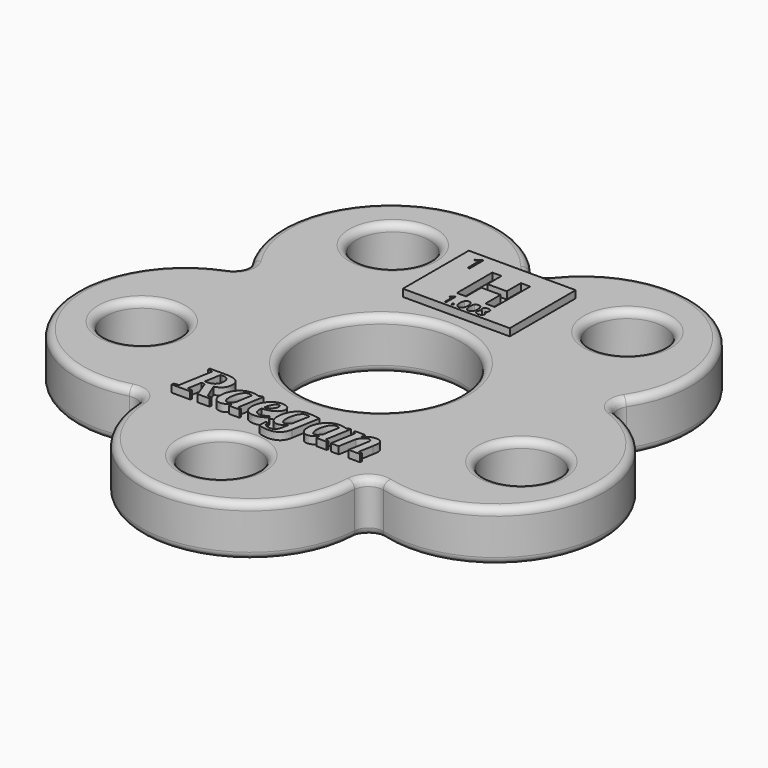
from build123d import *

# Parameters (mm, degrees)
F0_R         = 5
F0_R_2       = 11
F1_DEPTH     = 7
F2_R         = 2
F3_R         = 1
F4_W         = 14.733908698
F4_H         = 11.3537767902
F4_TEXT_SIZE = 8.3333333333
F5_DEPTH     = 1


# Not quite as in the source:
# - Text() gives the source's letters only with a copy of the font that has no kerning and outlines rounded to 1/6400 em; it was checked with that copy


with BuildPart() as f1:
    # F0 (on Top) → F1 (new body)
    with BuildSketch(Plane.XY):
        with BuildLine():
            ThreePointArc((24.0433357957, 7.8121533632), (22.041946961, 30.3381372891), (0, 25.2806593338))
            ThreePointArc((0, 25.2806593338), (-22.041946961, 30.3381372891), (-24.0433357957, 7.8121533632))
            ThreePointArc((-24.0433357957, 7.8121533632), (-35.6646193611, -11.5881372891), (-14.8595987247, -20.4524830301))
            ThreePointArc((-14.8595987247, -20.4524830301), (0, -37.5), (14.8595987247, -20.4524830301))
            ThreePointArc((14.8595987247, -20.4524830301), (35.6646193611, -11.5881372891), (24.0433357957, 7.8121533632))
        make_face()
        with Locations((-26.1540541981, -8.4979673453)):
            Circle(F0_R, mode=Mode.SUBTRACT)
        with Locations((0, -27.5)):
            Circle(F0_R, mode=Mode.SUBTRACT)
        with Locations((26.1540541981, -8.4979673453)):
            Circle(F0_R, mode=Mode.SUBTRACT)
        with Locations((-16.164094438, 22.2479673453)):
            Circle(F0_R, mode=Mode.SUBTRACT)
        Circle(F0_R_2, mode=Mode.SUBTRACT)
        with Locations((16.164094438, 22.2479673453)):
            Circle(F0_R, mode=Mode.SUBTRACT)
    extrude(amount=F1_DEPTH)

    # F2
    f2_edges = [f1.edges().sort_by_distance(p)[0] for p in [
        (14.859599, -20.452483, 3.5),
        (24.043336, 7.812153, 3.5),
        (0, 25.280659, 3.5),
        (-24.043336, 7.812153, 3.5),
        (-14.859599, -20.452483, 3.5),
    ]]
    fillet(f2_edges, radius=F2_R)

    # F3
    f3_edges = [f1.edges().sort_by_distance(p)[0] for p in [
        (35.664619, -11.588137, 7),
        (15.802257, -21.749941, 7),
        (25.568589, 8.307738, 7),
        (0, -37.5, 7),
        (22.041947, 30.338137, 7),
        (-15.802257, -21.749941, 7),
        (0, 26.884405, 7),
        (-35.664619, -11.588137, 7),
        (-22.041947, 30.338137, 7),
        (-25.568589, 8.307738, 7),
        (-31.154054, -8.497967, 7),
        (-5, -27.5, 7),
        (21.154054, -8.497967, 7),
        (-21.164094, 22.247967, 7),
        (-11, 0, 7),
        (11.164094, 22.247967, 7),
        (35.664619, -11.588137, 0),
        (15.802257, -21.749941, 0),
        (25.568589, 8.307738, 0),
        (0, -37.5, 0),
        (22.041947, 30.338137, 0),
        (-15.802257, -21.749941, 0),
        (0, 26.884405, 0),
        (-35.664619, -11.588137, 0),
        (-22.041947, 30.338137, 0),
        (-25.568589, 8.307738, 0),
        (-31.154054, -8.497967, 0),
        (-5, -27.5, 0),
        (21.154054, -8.497967, 0),
        (-21.164094, 22.247967, 0),
        (-11, 0, 0),
        (11.164094, 22.247967, 0),
    ]]
    fillet(f3_edges, radius=F3_R)

    # F4 (on face) → F5 (join)
    with BuildSketch(Plane.XY.offset(7)):
        with Locations((-0.4162131809, 19.1815658472)):
            Rectangle(F4_W, F4_H)
        with BuildLine():
            Line((-2.1715380596, 15.5983065148), (-2.1715380596, 13.9384558424))
            Line((-2.1715380596, 13.9384558424), (-2.3553604365, 13.9384558424))
            Line((-2.3553604365, 13.9384558424), (-2.3553604365, 15.1213128766))
            add(Edge.make_bspline(
                [(-2.3553604365, 15.1213128766), (-2.3553604365, 15.2691700059), (-2.3462783033, 15.4006792954)],
                knots=[0, 0, 0, 1, 1, 1], degree=2))
            add(Edge.make_bspline(
                [(-2.3462783033, 15.4006792954), (-2.3698918497, 15.3767024636), (-2.3994996041, 15.3507275625)],
                knots=[0, 0, 0, 1, 1, 1], degree=2))
            add(Edge.make_bspline(
                [(-2.3994996041, 15.3507275625), (-2.4291073585, 15.3247526614), (-2.6696022469, 15.1293051539)],
                knots=[0, 0, 0, 1, 1, 1], degree=2))
            Line((-2.6696022469, 15.1293051539), (-2.7695057126, 15.2586347314))
            Line((-2.7695057126, 15.2586347314), (-2.3302937488, 15.5983065148))
            Line((-2.3302937488, 15.5983065148), (-2.1715380596, 15.5983065148))
        make_face(mode=Mode.SUBTRACT)
        with BuildLine():
            add(Edge.make_bspline(
                [(-1.4433326158, 13.9411804824), (-1.4812959327, 13.9769640874), (-1.4812959327, 14.0587032866)],
                knots=[0, 0, 0, 1, 1, 1], degree=2))
            add(Edge.make_bspline(
                [(-1.4812959327, 14.0587032866), (-1.4812959327, 14.1349932059), (-1.4466021837, 14.1740463789)],
                knots=[0, 0, 0, 1, 1, 1], degree=2))
            add(Edge.make_bspline(
                [(-1.4466021837, 14.1740463789), (-1.4119084347, 14.2130995519), (-1.347243646, 14.2130995519)],
                knots=[0, 0, 0, 1, 1, 1], degree=2))
            add(Edge.make_bspline(
                [(-1.347243646, 14.2130995519), (-1.2814890013, 14.2130995519), (-1.2446155403, 14.1740463789)],
                knots=[0, 0, 0, 1, 1, 1], degree=2))
            add(Edge.make_bspline(
                [(-1.2446155403, 14.1740463789), (-1.2077420793, 14.1349932059), (-1.2077420793, 14.0587032866)],
                knots=[0, 0, 0, 1, 1, 1], degree=2))
            add(Edge.make_bspline(
                [(-1.2077420793, 14.0587032866), (-1.2077420793, 13.9849563647), (-1.2451604683, 13.945176621)],
                knots=[0, 0, 0, 1, 1, 1], degree=2))
            add(Edge.make_bspline(
                [(-1.2451604683, 13.945176621), (-1.2825788573, 13.9053968774), (-1.347243646, 13.9053968774)],
                knots=[0, 0, 0, 1, 1, 1], degree=2))
            add(Edge.make_bspline(
                [(-1.347243646, 13.9053968774), (-1.4053692988, 13.9053968774), (-1.4433326158, 13.9411804824)],
                knots=[0, 0, 0, 1, 1, 1], degree=2))
        make_face(mode=Mode.SUBTRACT)
        with BuildLine():
            add(Edge.make_bspline(
                [(0.0383266023, 15.405220362), (0.1785547397, 15.1859776654), (0.1785547397, 14.7707425333)],
                knots=[0, 0, 0, 1, 1, 1], degree=2))
            add(Edge.make_bspline(
                [(0.1785547397, 14.7707425333), (0.1785547397, 14.3402494173), (0.0428676689, 14.127909142)],
                knots=[0, 0, 0, 1, 1, 1], degree=2))
            add(Edge.make_bspline(
                [(0.0428676689, 14.127909142), (-0.0928194018, 13.9155688667), (-0.3721858205, 13.9155688667)],
                knots=[0, 0, 0, 1, 1, 1], degree=2))
            add(Edge.make_bspline(
                [(-0.3721858205, 13.9155688667), (-0.6399271086, 13.9155688667), (-0.779610318, 14.1329951366)],
                knots=[0, 0, 0, 1, 1, 1], degree=2))
            add(Edge.make_bspline(
                [(-0.779610318, 14.1329951366), (-0.9192935274, 14.3504214066), (-0.9192935274, 14.7707425333)],
                knots=[0, 0, 0, 1, 1, 1], degree=2))
            add(Edge.make_bspline(
                [(-0.9192935274, 14.7707425333), (-0.9192935274, 15.2041419319), (-0.7841513846, 15.4143024952)],
                knots=[0, 0, 0, 1, 1, 1], degree=2))
            add(Edge.make_bspline(
                [(-0.7841513846, 15.4143024952), (-0.6490092419, 15.6244630586), (-0.3721858205, 15.6244630586)],
                knots=[0, 0, 0, 1, 1, 1], degree=2))
            add(Edge.make_bspline(
                [(-0.3721858205, 15.6244630586), (-0.101901535, 15.6244630586), (0.0383266023, 15.405220362)],
                knots=[0, 0, 0, 1, 1, 1], degree=2))
        make_face(mode=Mode.SUBTRACT)
        with BuildLine():
            Line((-5.1220975915, 24.0717205949), (-5.1220975915, 21.6852203012))
            Line((-5.1220975915, 21.6852203012), (-5.3863937501, 21.6852203012))
            Line((-5.3863937501, 21.6852203012), (-5.3863937501, 23.385908626))
            add(Edge.make_bspline(
                [(-5.3863937501, 23.385908626), (-5.3863937501, 23.5984946667), (-5.3733356395, 23.7875761082)],
                knots=[0, 0, 0, 1, 1, 1], degree=2))
            add(Edge.make_bspline(
                [(-5.3733356395, 23.7875761082), (-5.4072867271, 23.7531026962), (-5.4498561676, 23.7157564999)],
                knots=[0, 0, 0, 1, 1, 1], degree=2))
            add(Edge.make_bspline(
                [(-5.4498561676, 23.7157564999), (-5.4924256082, 23.6784103035), (-5.8382043769, 23.3973997634)],
                knots=[0, 0, 0, 1, 1, 1], degree=2))
            Line((-5.8382043769, 23.3973997634), (-5.9818435936, 23.5833472584))
            Line((-5.9818435936, 23.5833472584), (-5.3503533648, 24.0717205949))
            Line((-5.3503533648, 24.0717205949), (-5.1220975915, 24.0717205949))
        make_face(mode=Mode.SUBTRACT)
        with BuildLine():
            add(Edge.make_bspline(
                [(1.3675876245, 15.405220362), (1.5078157618, 15.1859776654), (1.5078157618, 14.7707425333)],
                knots=[0, 0, 0, 1, 1, 1], degree=2))
            add(Edge.make_bspline(
                [(1.5078157618, 14.7707425333), (1.5078157618, 14.3402494173), (1.3721286911, 14.127909142)],
                knots=[0, 0, 0, 1, 1, 1], degree=2))
            add(Edge.make_bspline(
                [(1.3721286911, 14.127909142), (1.2364416204, 13.9155688667), (0.9570752017, 13.9155688667)],
                knots=[0, 0, 0, 1, 1, 1], degree=2))
            add(Edge.make_bspline(
                [(0.9570752017, 13.9155688667), (0.6893339135, 13.9155688667), (0.5496507042, 14.1329951366)],
                knots=[0, 0, 0, 1, 1, 1], degree=2))
            add(Edge.make_bspline(
                [(0.5496507042, 14.1329951366), (0.4099674948, 14.3504214066), (0.4099674948, 14.7707425333)],
                knots=[0, 0, 0, 1, 1, 1], degree=2))
            add(Edge.make_bspline(
                [(0.4099674948, 14.7707425333), (0.4099674948, 15.2041419319), (0.5451096375, 15.4143024952)],
                knots=[0, 0, 0, 1, 1, 1], degree=2))
            add(Edge.make_bspline(
                [(0.5451096375, 15.4143024952), (0.6802517803, 15.6244630586), (0.9570752017, 15.6244630586)],
                knots=[0, 0, 0, 1, 1, 1], degree=2))
            add(Edge.make_bspline(
                [(0.9570752017, 15.6244630586), (1.2273594871, 15.6244630586), (1.3675876245, 15.405220362)],
                knots=[0, 0, 0, 1, 1, 1], degree=2))
        make_face(mode=Mode.SUBTRACT)
        with BuildLine():
            add(Edge.make_bspline(
                [(1.9292267445, 15.5147508889), (2.0625524606, 15.6219200613), (2.2863362238, 15.6219200613)],
                knots=[0, 0, 0, 1, 1, 1], degree=2))
            add(Edge.make_bspline(
                [(2.2863362238, 15.6219200613), (2.513389555, 15.6219200613), (2.6461703431, 15.5163856729)],
                knots=[0, 0, 0, 1, 1, 1], degree=2))
            add(Edge.make_bspline(
                [(2.6461703431, 15.5163856729), (2.7789511312, 15.4108512846), (2.7789511312, 15.2248491957)],
                knots=[0, 0, 0, 1, 1, 1], degree=2))
            add(Edge.make_bspline(
                [(2.7789511312, 15.2248491957), (2.7789511312, 15.1020587542), (2.7030244972, 15.0010654324)],
                knots=[0, 0, 0, 1, 1, 1], degree=2))
            add(Edge.make_bspline(
                [(2.7030244972, 15.0010654324), (2.6270978633, 14.9000721107), (2.4599866115, 14.8172430555)],
                knots=[0, 0, 0, 1, 1, 1], degree=2))
            add(Edge.make_bspline(
                [(2.4599866115, 14.8172430555), (2.661973255, 14.7206091577), (2.7471636648, 14.6145298414)],
                knots=[0, 0, 0, 1, 1, 1], degree=2))
            add(Edge.make_bspline(
                [(2.7471636648, 14.6145298414), (2.8323540747, 14.5084505251), (2.8323540747, 14.3685856731)],
                knots=[0, 0, 0, 1, 1, 1], degree=2))
            add(Edge.make_bspline(
                [(2.8323540747, 14.3685856731), (2.8323540747, 14.1622396057), (2.6881297987, 14.0389042362)],
                knots=[0, 0, 0, 1, 1, 1], degree=2))
            add(Edge.make_bspline(
                [(2.6881297987, 14.0389042362), (2.5439055227, 13.9155688667), (2.2932386451, 13.9155688667)],
                knots=[0, 0, 0, 1, 1, 1], degree=2))
            add(Edge.make_bspline(
                [(2.2932386451, 13.9155688667), (2.0276770689, 13.9155688667), (1.8845426489, 14.0320018149)],
                knots=[0, 0, 0, 1, 1, 1], degree=2))
            add(Edge.make_bspline(
                [(1.8845426489, 14.0320018149), (1.741408229, 14.1484347631), (1.741408229, 14.3620465371)],
                knots=[0, 0, 0, 1, 1, 1], degree=2))
            add(Edge.make_bspline(
                [(1.741408229, 14.3620465371), (1.741408229, 14.6468622358), (2.0887090044, 14.8059812103)],
                knots=[0, 0, 0, 1, 1, 1], degree=2))
            add(Edge.make_bspline(
                [(2.0887090044, 14.8059812103), (1.9321330272, 14.8942595454), (1.8640170278, 14.9970692938)],
                knots=[0, 0, 0, 1, 1, 1], degree=2))
            add(Edge.make_bspline(
                [(1.8640170278, 14.9970692938), (1.7959010284, 15.0998790422), (1.7959010284, 15.2270289077)],
                knots=[0, 0, 0, 1, 1, 1], degree=2))
            add(Edge.make_bspline(
                [(1.7959010284, 15.2270289077), (1.7959010284, 15.4075817166), (1.9292267445, 15.5147508889)],
                knots=[0, 0, 0, 1, 1, 1], degree=2))
        make_face(mode=Mode.SUBTRACT)
        Polygon((2.5982840531, 16.3463894278), (1.3195982261, 16.3463894278), (1.3195982261, 18.9647829652), (-1.3417880018, 18.9647829652), (-1.3417880018, 16.3463894278), (-2.6204738289, 16.3463894278), (-2.6204738289, 22.4527383394), (-1.3417880018, 22.4527383394), (-1.3417880018, 20.0215710348), (1.3195982261, 20.0215710348), (1.3195982261, 22.4527383394), (2.5982840531, 22.4527383394), align=None, mode=Mode.SUBTRACT)
        with Locations((-13.2591145833, -19.4611851107)):
            Text('Raegan', F4_TEXT_SIZE, font='Tinos', font_style=FontStyle.BOLDITALIC, text_align=(TextAlign.LEFT, TextAlign.BOTTOM))
    extrude(amount=F5_DEPTH)


solid = f1.part
